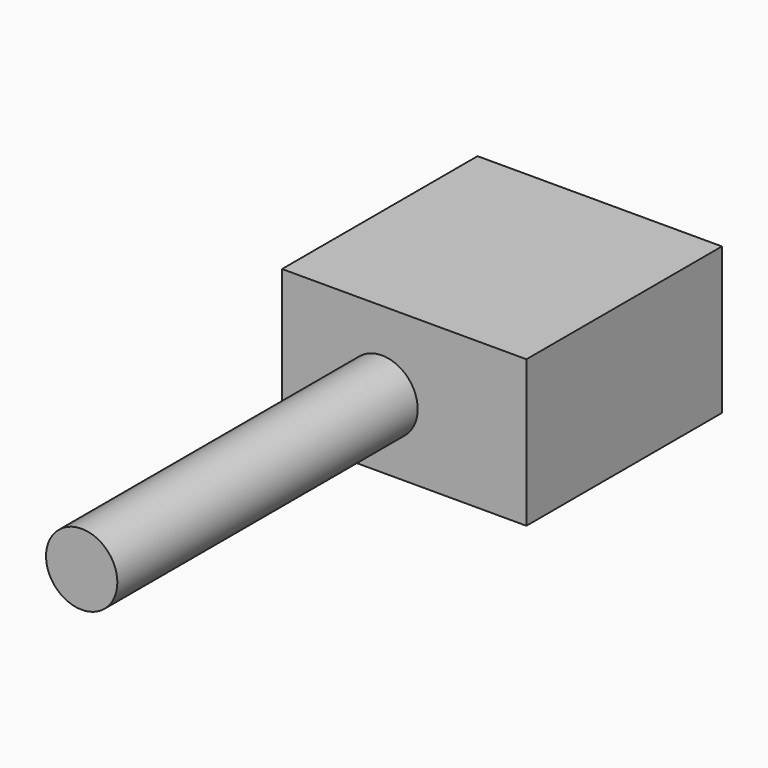
from build123d import *

# Parameters (mm, degrees)
F1_W     = 50
F1_H     = 30
F2_DEPTH = 50
F3_R     = 7.2976744804
F4_DEPTH = 76.8214575
F5_DEPTH = 116.5


# Not quite as in the source:
# - an extrude ends at something that could not be found from the text; its depth is read off the source's solid


with BuildPart() as f2:
    # F1 (on Right) → F2 (new body)
    with BuildSketch(Plane.YZ):
        with Locations((25, 15)):
            Rectangle(F1_W, F1_H)
    extrude(amount=F2_DEPTH)

    # F3 (on face) → F4 (join, through all)
    with BuildSketch(Plane.XZ):
        with Locations((20.4548016191, 13.7891862541)):
            Circle(F3_R)
    extrude(amount=F4_DEPTH)

    # F5 (add): a face of the model
    f5_faces = [f2.faces().sort_by_distance(p)[0] for p in [
        (20.4548016191, -76.8214575, 13.7891862541),
    ]]
    extrude(f5_faces, amount=-F5_DEPTH)


solid = f2.part
